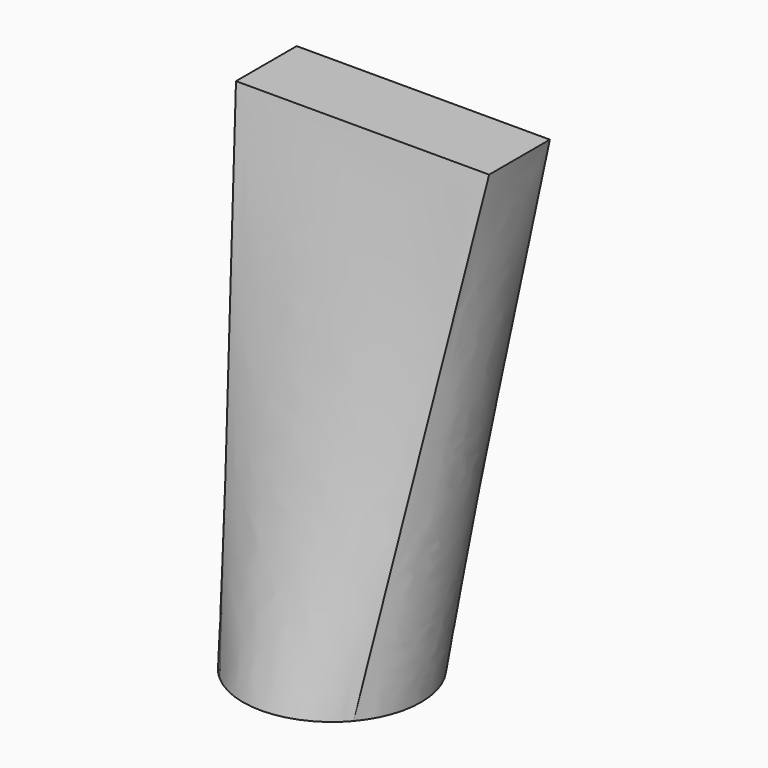
from build123d import *

# Parameters (mm, degrees)
F2_W = 81.4404524863
F2_H = 24.4130641222


# Not quite as in the source:
# - the arcs of a loft's sections are written as splines that run evenly, so that the points pair up as in the source's solid


with BuildPart() as f3:
    # F2 (on offset) → F3 section 0
    with BuildSketch(Plane.XY.offset(152.4)):
        with Locations((4.8635397106, 18.405161798)):
            Rectangle(F2_W, F2_H)
    # F0 (on Top) → F3 section 1
    with BuildSketch(Plane.XY):
        with BuildLine():
            add(Edge.make_bspline(
                [(-21.7946915268, 18.6066390761), (-23.0124932066, 17.1801798513), (-24.089774277, 15.6338158679), (-25.9220014219, 12.3605528028), (-26.6769021911, 10.6337346588), (-27.8353416598, 7.0659166419), (-28.2388517146, 5.2250049902), (-28.6789853279, 1.4997412671), (-28.7155980033, -0.3845186899), (-28.4205116733, -4.1240683236), (-28.0888199645, -5.9792655325), (-27.0698536934, -9.5893922813), (-26.382604327, -11.3442325538), (-24.6789164171, -14.6862012715), (-23.6625200007, -16.27324708), (-21.3395822229, -19.2186277829), (-20.0330983008, -20.5768898471), (-18.6066390761, -21.7946915268)],
                knots=[0, 0, 0, 0, 0.125, 0.125, 0.25, 0.25, 0.375, 0.375, 0.5, 0.5, 0.625, 0.625, 0.75, 0.75, 0.875, 0.875, 1, 1, 1, 1], degree=3))
            add(Edge.make_bspline(
                [(-18.6066390761, -21.7946915268), (-17.1801798513, -23.0124932066), (-15.6338158679, -24.089774277), (-12.3605528028, -25.9220014219), (-10.6337346588, -26.6769021911), (-7.0659166419, -27.8353416598), (-5.2250049902, -28.2388517146), (-1.4997412671, -28.6789853279), (0.3845186899, -28.7155980033), (4.1240683236, -28.4205116733), (5.9792655325, -28.0888199645), (9.5893922813, -27.0698536934), (11.3442325538, -26.382604327), (14.6862012715, -24.6789164171), (16.27324708, -23.6625200007), (19.2186277829, -21.3395822229), (20.5768898471, -20.0330983008), (21.7946915268, -18.6066390761)],
                knots=[0, 0, 0, 0, 0.125, 0.125, 0.25, 0.25, 0.375, 0.375, 0.5, 0.5, 0.625, 0.625, 0.75, 0.75, 0.875, 0.875, 1, 1, 1, 1], degree=3))
            add(Edge.make_bspline(
                [(21.7946915268, -18.6066390761), (23.0124932066, -17.1801798513), (24.089774277, -15.6338158679), (25.9220014219, -12.3605528028), (26.6769021911, -10.6337346588), (27.8353416598, -7.0659166419), (28.2388517146, -5.2250049902), (28.6789853279, -1.4997412671), (28.7155980033, 0.3845186899), (28.4205116733, 4.1240683236), (28.0888199645, 5.9792655325), (27.0698536934, 9.5893922813), (26.382604327, 11.3442325538), (24.6789164171, 14.6862012715), (23.6625200007, 16.27324708), (21.3395822229, 19.2186277829), (20.0330983008, 20.5768898471), (18.6066390761, 21.7946915268)],
                knots=[0, 0, 0, 0, 0.125, 0.125, 0.25, 0.25, 0.375, 0.375, 0.5, 0.5, 0.625, 0.625, 0.75, 0.75, 0.875, 0.875, 1, 1, 1, 1], degree=3))
            add(Edge.make_bspline(
                [(18.6066390761, 21.7946915268), (17.1801798513, 23.0124932066), (15.6338158679, 24.089774277), (12.3605528028, 25.9220014219), (10.6337346588, 26.6769021911), (7.0659166419, 27.8353416598), (5.2250049902, 28.2388517146), (1.4997412671, 28.6789853279), (-0.3845186899, 28.7155980033), (-4.1240683236, 28.4205116733), (-5.9792655325, 28.0888199645), (-9.5893922813, 27.0698536934), (-11.3442325538, 26.382604327), (-14.6862012715, 24.6789164171), (-16.27324708, 23.6625200007), (-19.2186277829, 21.3395822229), (-20.5768898471, 20.0330983008), (-21.7946915268, 18.6066390761)],
                knots=[0, 0, 0, 0, 0.125, 0.125, 0.25, 0.25, 0.375, 0.375, 0.5, 0.5, 0.625, 0.625, 0.75, 0.75, 0.875, 0.875, 1, 1, 1, 1], degree=3))
        make_face()
    loft(ruled=True)


solid = f3.part
